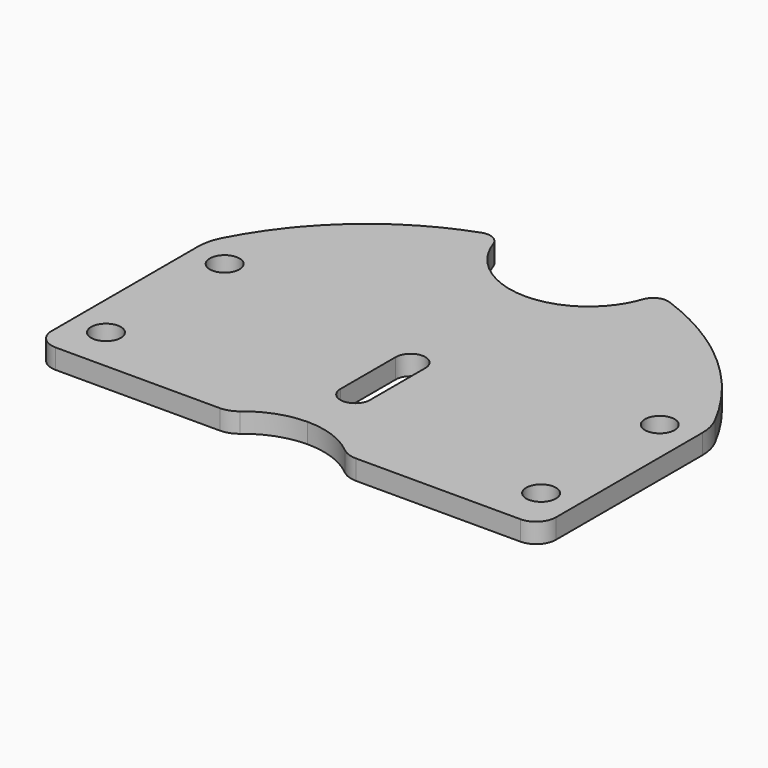
from build123d import *

# Parameters (mm, degrees)
F0_R     = 1.5
F1_DEPTH = 2


# Not quite as in the source:
# - a feature names something its author has since deleted; it is built from what else it names


with BuildPart() as f1:
    # F0 (on Top) → F1 (new body)
    with BuildSketch(Plane.XY):
        with BuildLine():
            Line((-61.8704294452, 175.1948396463), (-53.8704294452, 175.1948396463))
            Line((-53.8704294452, 175.1948396463), (-53.8704294452, 185.547974161))
            ThreePointArc((-53.8704294452, 185.547974161), (-57.1946545112, 183.1877510697), (-58.3269518777, 187.1042581875))
            ThreePointArc((-58.3269518777, 187.1042581875), (-59.9354051762, 184.8644644288), (-61.3162125777, 182.4775901096))
            ThreePointArc((-61.3162125777, 182.4775901096), (-61.7299003867, 181.366665728), (-61.8704294452, 180.1895751756))
            Line((-61.8704294452, 180.1895751756), (-61.8704294452, 175.1948396463))
        make_face()
        with Locations((-58.3704294452, 179.1948396463)):
            Circle(F0_R, mode=Mode.SUBTRACT)
        with BuildLine():
            ThreePointArc((-58.3269518777, 187.1042581875), (-57.1946545112, 183.1877510697), (-53.8704294452, 185.547974161))
            ThreePointArc((-53.8704294452, 185.547974161), (-54.6026624922, 187.315741114), (-56.3704294452, 188.047974161))
            ThreePointArc((-56.3704294452, 188.047974161), (-57.4565440648, 187.7997190473), (-58.3269518777, 187.1042581875))
        make_face()
        with BuildLine():
            Line((-18.8704294452, 175.1948396463), (-10.8704294452, 175.1948396463))
            Line((-10.8704294452, 175.1948396463), (-10.8704294452, 180.1895751756))
            ThreePointArc((-10.8704294452, 180.1895751756), (-11.0109585037, 181.366665728), (-11.4246463127, 182.4775901096))
            ThreePointArc((-11.4246463127, 182.4775901096), (-12.8054541473, 184.8644650992), (-14.4139080064, 187.1042594368))
            ThreePointArc((-14.4139080064, 187.1042594368), (-14.010206617, 186.3721999805), (-13.8704294452, 185.547974161))
            ThreePointArc((-13.8704294452, 185.547974161), (-16.3704294452, 183.047974161), (-18.8704294452, 185.547974161))
            Line((-18.8704294452, 185.547974161), (-18.8704294452, 175.1948396463))
        make_face()
        with Locations((-14.3704294452, 179.1948396463)):
            Circle(F0_R, mode=Mode.SUBTRACT)
        with BuildLine():
            ThreePointArc((-16.3704294452, 188.047974161), (-18.1381963982, 187.315741114), (-18.8704294452, 185.547974161))
            ThreePointArc((-18.8704294452, 185.547974161), (-16.3704294452, 183.047974161), (-13.8704294452, 185.547974161))
            ThreePointArc((-13.8704294452, 185.547974161), (-14.010206617, 186.3721999805), (-14.4139080064, 187.1042594368))
            ThreePointArc((-14.4139080064, 187.1042594368), (-15.2843155445, 187.7997193941), (-16.3704294452, 188.047974161))
        make_face()
        with BuildLine():
            Line((-36.3704294452, 166.6948396463), (-36.3704294452, 165.1948396463))
            Line((-36.3704294452, 165.1948396463), (-23.8704294452, 165.1948396463))
            ThreePointArc((-23.8704294452, 165.1948396463), (-20.3348955393, 166.6593057403), (-18.8704294452, 170.1948396463))
            Line((-18.8704294452, 170.1948396463), (-18.8704294452, 175.1948396463))
            Line((-18.8704294452, 175.1948396463), (-34.8704294452, 175.1948396463))
            Line((-34.8704294452, 175.1948396463), (-34.8704294452, 168.1948396463))
            ThreePointArc((-34.8704294452, 168.1948396463), (-35.3097692734, 167.1341794745), (-36.3704294452, 166.6948396463))
        make_face()
        with BuildLine():
            Line((-48.8704294452, 165.1948396463), (-36.3704294452, 165.1948396463))
            Line((-36.3704294452, 165.1948396463), (-36.3704294452, 166.6948396463))
            ThreePointArc((-36.3704294452, 166.6948396463), (-37.431089617, 167.1341794745), (-37.8704294452, 168.1948396463))
            Line((-37.8704294452, 168.1948396463), (-37.8704294452, 175.1948396463))
            Line((-37.8704294452, 175.1948396463), (-53.8704294452, 175.1948396463))
            Line((-53.8704294452, 175.1948396463), (-53.8704294452, 170.1948396463))
            ThreePointArc((-53.8704294452, 170.1948396463), (-52.4059633511, 166.6593057403), (-48.8704294452, 165.1948396463))
        make_face()
        with BuildLine():
            Line((-34.8704294452, 175.1948396463), (-18.8704294452, 175.1948396463))
            Line((-18.8704294452, 175.1948396463), (-18.8704294452, 185.547974161))
            Line((-18.8704294452, 185.547974161), (-18.8704294452, 188.047974161))
            Line((-18.8704294452, 188.047974161), (-53.8704294452, 188.047974161))
            Line((-53.8704294452, 188.047974161), (-53.8704294452, 185.547974161))
            Line((-53.8704294452, 185.547974161), (-53.8704294452, 175.1948396463))
            Line((-53.8704294452, 175.1948396463), (-37.8704294452, 175.1948396463))
            ThreePointArc((-37.8704294452, 175.1948396463), (-36.3704294452, 176.6948396463), (-34.8704294452, 175.1948396463))
        make_face()
        with BuildLine():
            ThreePointArc((-41.6596574736, 160.2762349793), (-39.1836561071, 161.7003703018), (-36.3704294452, 162.1948396463))
            Line((-36.3704294452, 162.1948396463), (-36.3704294452, 165.1948396463))
            Line((-36.3704294452, 165.1948396463), (-48.8704294452, 165.1948396463))
            ThreePointArc((-48.8704294452, 165.1948396463), (-52.4059633511, 166.6593057403), (-53.8704294452, 170.1948396463))
            Line((-53.8704294452, 170.1948396463), (-53.8704294452, 175.1948396463))
            Line((-53.8704294452, 175.1948396463), (-61.8704294452, 175.1948396463))
            Line((-61.8704294452, 175.1948396463), (-61.8704294452, 161.6948396463))
            ThreePointArc((-61.8704294452, 161.6948396463), (-61.2846430076, 160.2806260839), (-59.8704294452, 159.6948396463))
            Line((-59.8704294452, 159.6948396463), (-43.2624538212, 159.6948396463))
            ThreePointArc((-43.2624538212, 159.6948396463), (-45.0302207742, 163.9626065992), (-40.7624538212, 162.1948396463))
            ThreePointArc((-40.7624538212, 162.1948396463), (-40.997835656, 161.13582852), (-41.6596574736, 160.2762349793))
        make_face()
        with Locations((-58.3704294452, 164.1948396463)):
            Circle(F0_R, mode=Mode.SUBTRACT)
        with BuildLine():
            ThreePointArc((-43.2624538212, 159.6948396463), (-42.4099609085, 159.8446788361), (-41.6596574736, 160.2762349793))
            ThreePointArc((-41.6596574736, 160.2762349793), (-40.997835656, 161.13582852), (-40.7624538212, 162.1948396463))
            ThreePointArc((-40.7624538212, 162.1948396463), (-45.0302207742, 163.9626065992), (-43.2624538212, 159.6948396463))
        make_face()
        with BuildLine():
            ThreePointArc((-56.3704294452, 188.047974161), (-54.6026624922, 187.315741114), (-53.8704294452, 185.547974161))
            Line((-53.8704294452, 185.547974161), (-53.8704294452, 188.047974161))
            Line((-53.8704294452, 188.047974161), (-56.3704294452, 188.047974161))
        make_face()
        with BuildLine():
            Line((-18.8704294452, 188.047974161), (-18.8704294452, 185.547974161))
            ThreePointArc((-18.8704294452, 185.547974161), (-18.1381963982, 187.315741114), (-16.3704294452, 188.047974161))
            Line((-16.3704294452, 188.047974161), (-18.8704294452, 188.047974161))
        make_face()
        with BuildLine():
            ThreePointArc((-26.9784050691, 162.1948396463), (-27.7106381162, 160.4270726933), (-29.4784050691, 159.6948396463))
            Line((-29.4784050691, 159.6948396463), (-12.8704294452, 159.6948396463))
            ThreePointArc((-12.8704294452, 159.6948396463), (-11.4562158828, 160.2806260839), (-10.8704294452, 161.6948396463))
            Line((-10.8704294452, 161.6948396463), (-10.8704294452, 175.1948396463))
            Line((-10.8704294452, 175.1948396463), (-18.8704294452, 175.1948396463))
            Line((-18.8704294452, 175.1948396463), (-18.8704294452, 170.1948396463))
            ThreePointArc((-18.8704294452, 170.1948396463), (-20.3348955393, 166.6593057403), (-23.8704294452, 165.1948396463))
            Line((-23.8704294452, 165.1948396463), (-36.3704294452, 165.1948396463))
            Line((-36.3704294452, 165.1948396463), (-36.3704294452, 162.1948396463))
            ThreePointArc((-36.3704294452, 162.1948396463), (-33.557202708, 161.7003702745), (-31.0812012938, 160.2762348766))
            ThreePointArc((-31.0812012938, 160.2762348766), (-30.5374162679, 164.4594577776), (-26.9784050691, 162.1948396463))
        make_face()
        with Locations((-14.3704294452, 164.1948396463)):
            Circle(F0_R, mode=Mode.SUBTRACT)
        with BuildLine():
            ThreePointArc((-31.0812012938, 160.2762348766), (-30.3308979066, 159.8446788088), (-29.4784050691, 159.6948396463))
            ThreePointArc((-29.4784050691, 159.6948396463), (-27.7106381162, 160.4270726933), (-26.9784050691, 162.1948396463))
            ThreePointArc((-26.9784050691, 162.1948396463), (-30.5374162679, 164.4594577776), (-31.0812012938, 160.2762348766))
        make_face()
        with BuildLine():
            Line((-53.8704294452, 188.047974161), (-18.8704294452, 188.047974161))
            Line((-18.8704294452, 188.047974161), (-18.8704294452, 191.5679000418))
            ThreePointArc((-18.8704294452, 191.5679000418), (-19.871628172, 192.3307748764), (-20.9060372255, 193.047974161))
            Line((-20.9060372255, 193.047974161), (-29.8583912725, 193.047974161))
            ThreePointArc((-29.8583912725, 193.047974161), (-36.3704294452, 189.6948396463), (-42.8824676178, 193.047974161))
            Line((-42.8824676178, 193.047974161), (-51.8348216648, 193.047974161))
            ThreePointArc((-51.8348216648, 193.047974161), (-52.8692307184, 192.3307748764), (-53.8704294452, 191.5679000418))
            Line((-53.8704294452, 191.5679000418), (-53.8704294452, 188.047974161))
        make_face()
        with BuildLine():
            Line((-56.3704294452, 188.047974161), (-53.8704294452, 188.047974161))
            Line((-53.8704294452, 188.047974161), (-53.8704294452, 191.5679000418))
            ThreePointArc((-53.8704294452, 191.5679000418), (-55.7861337119, 189.8913117759), (-57.5419746752, 188.047974161))
            Line((-57.5419746752, 188.047974161), (-56.3704294452, 188.047974161))
        make_face()
        with BuildLine():
            Line((-18.8704294452, 191.5679000418), (-18.8704294452, 188.047974161))
            Line((-18.8704294452, 188.047974161), (-16.3704294452, 188.047974161))
            Line((-16.3704294452, 188.047974161), (-15.1988842152, 188.047974161))
            ThreePointArc((-15.1988842152, 188.047974161), (-16.9547251785, 189.8913117759), (-18.8704294452, 191.5679000418))
        make_face()
        with BuildLine():
            ThreePointArc((-58.3269518777, 187.1042581875), (-57.4565440648, 187.7997190473), (-56.3704294452, 188.047974161))
            Line((-56.3704294452, 188.047974161), (-57.5419746752, 188.047974161))
            ThreePointArc((-57.5419746752, 188.047974161), (-57.939625189, 187.5804098217), (-58.3269518777, 187.1042581875))
        make_face()
        with BuildLine():
            Line((-15.1988842152, 188.047974161), (-16.3704294452, 188.047974161))
            ThreePointArc((-16.3704294452, 188.047974161), (-15.2843155445, 187.7997193941), (-14.4139080064, 187.1042594368))
            ThreePointArc((-14.4139080064, 187.1042594368), (-14.8012342118, 187.5804104353), (-15.1988842152, 188.047974161))
        make_face()
        with BuildLine():
            Line((-29.8583912725, 193.047974161), (-20.9060372255, 193.047974161))
            ThreePointArc((-20.9060372255, 193.047974161), (-23.799669125, 194.7209543402), (-26.8717251154, 196.0379358287))
            ThreePointArc((-26.8717251154, 196.0379358287), (-26.1524301853, 195.489141652), (-25.8795767704, 194.6265228146))
            ThreePointArc((-25.8795767704, 194.6265228146), (-27.6251244235, 193.1467571743), (-28.7991852371, 195.1109934548))
            ThreePointArc((-28.7991852371, 195.1109934548), (-29.2536378362, 194.0408996913), (-29.8583912725, 193.047974161))
        make_face()
        with BuildLine():
            ThreePointArc((-25.8795767704, 194.6265228146), (-26.1524301853, 195.489141652), (-26.8717251154, 196.0379358287))
            ThreePointArc((-26.8717251154, 196.0379358287), (-28.0296772719, 195.97832507), (-28.7991852371, 195.1109934548))
            ThreePointArc((-28.7991852371, 195.1109934548), (-27.6251244235, 193.1467571743), (-25.8795767704, 194.6265228146))
        make_face()
        with BuildLine():
            ThreePointArc((-43.9416738286, 195.1109939684), (-44.7111817722, 195.978325144), (-45.8691335854, 196.037935897))
            ThreePointArc((-45.8691335854, 196.037935897), (-46.2239010399, 193.3993762875), (-43.86128212, 194.6265228146))
            ThreePointArc((-43.86128212, 194.6265228146), (-43.8815165242, 194.8720707354), (-43.9416738286, 195.1109939684))
        make_face()
        with BuildLine():
            ThreePointArc((-45.8691335854, 196.037935897), (-48.9411896753, 194.7209543853), (-51.8348216648, 193.047974161))
            Line((-51.8348216648, 193.047974161), (-42.8824676178, 193.047974161))
            ThreePointArc((-42.8824676178, 193.047974161), (-43.4872211781, 194.0408999327), (-43.9416738286, 195.1109939684))
            ThreePointArc((-43.9416738286, 195.1109939684), (-43.8815165242, 194.8720707354), (-43.86128212, 194.6265228146))
            ThreePointArc((-43.86128212, 194.6265228146), (-46.2239010399, 193.3993762875), (-45.8691335854, 196.037935897))
        make_face()
    extrude(amount=F1_DEPTH)


solid = f1.part
